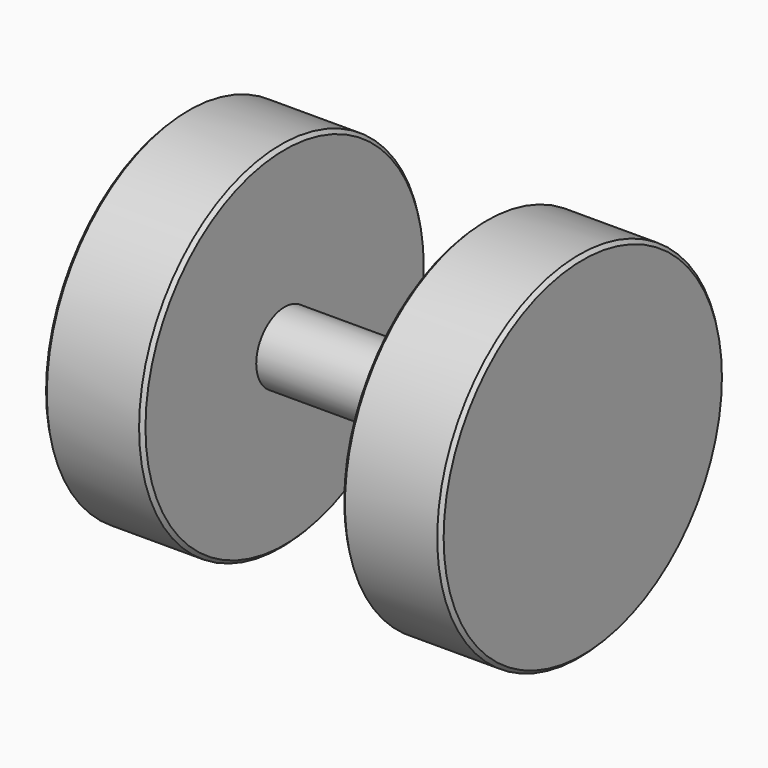
from build123d import *

# Parameters (mm, degrees)
F0_R     = 25
F1_DEPTH = 14
F2_R     = 5
F3_DEPTH = 28
F4_R     = 25
F5_DEPTH = 14
F6_SIZE  = 0.5


with BuildPart() as f1:
    # F0 (on Right) → F1 (new body)
    with BuildSketch(Plane.YZ):
        Circle(F0_R)
    extrude(amount=F1_DEPTH)

    # F2 (on face) → F3 (join)
    with BuildSketch(Plane(origin=(0, 0, 0), x_dir=(0, -1, 0), z_dir=(-1, 0, 0))):
        Circle(F2_R)
    extrude(amount=F3_DEPTH)

    # F4 (on face) → F5 (join)
    with BuildSketch(Plane(origin=(-28, 0, 0), x_dir=(0, -1, 0), z_dir=(-1, 0, 0))):
        Circle(F4_R)
    extrude(amount=F5_DEPTH)

    # F6
    f6_edges = [f1.edges().sort_by_distance(p)[0] for p in [
        (14, -25, 0),
        (0, -25, 0),
        (-35, -25, 0),
        (-28, 25, 0),
        (-42, 25, 0),
    ]]
    chamfer(f6_edges, length=F6_SIZE)


solid = f1.part
